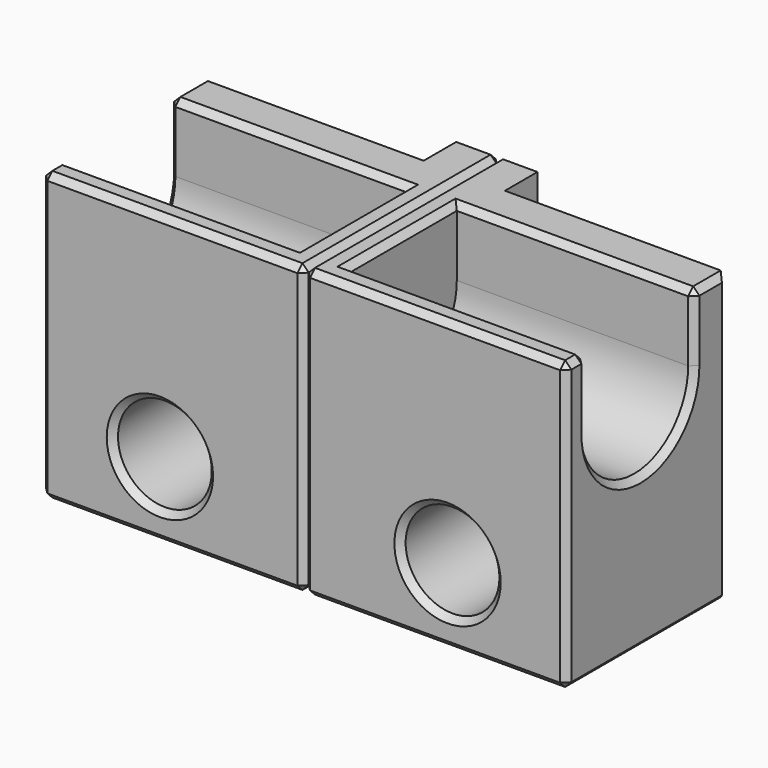
from build123d import *

# Parameters (mm, degrees)
F6_R      = 7.5
F6_R_2    = 4
F6_W      = 4
F6_H      = 4
F7_DEPTH  = 29.6
F8_DEPTH  = 2.5
F9_DEPTH  = 10
F10_DEPTH = 2.5
F12_DEPTH = 38
F14_W     = 7.5
F14_H     = 20
F15_DEPTH = 2.5
F16_R     = 7.5
F16_R_2   = 4
F17_DEPTH = 21.6
F18_SIZE  = 1


with BuildPart() as f7:
    # F6 (on Front) → F7 (new body)
    with BuildSketch(Plane.XZ):
        Polygon((0, -12), (-19, -12), (-19, -34), (0, -34), (15, -34), (15, -12), align=None)
        with Locations((0, -26)):
            Circle(F6_R, mode=Mode.SUBTRACT)
        Polygon((15, 8), (0, 8), (-19, 8), (-19, -12), (0, -12), (15, -12), align=None)
        Circle(F6_R_2, mode=Mode.SUBTRACT)
        with Locations((0, -26)):
            Circle(F6_R)
        with Locations((0, -26)):
            Circle(F6_R_2, mode=Mode.SUBTRACT)
        Polygon((-19, -12), (-19, 8), (-23, 8), (-23, -34), (-19, -34), align=None)
        Polygon((19, 8), (15, 8), (15, -12), (15, -34), (19, -34), align=None)
        Polygon((0, -34), (-19, -34), (-19, -38), (15, -38), (15, -34), align=None)
        Circle(F6_R_2)
        with Locations((-21, -36)):
            Rectangle(F6_W, F6_H)
        with Locations((17, -36)):
            Rectangle(F6_W, F6_H)
    extrude(amount=F7_DEPTH)

    # F6 (on Front) → F8 (join)
    with BuildSketch(Plane.XZ):
        Polygon((15, 8), (0, 8), (-19, 8), (-19, -12), (0, -12), (15, -12), align=None)
        Circle(F6_R_2, mode=Mode.SUBTRACT)
        Circle(F6_R_2)
    extrude(amount=-F8_DEPTH)

    # F6 (on Front) → F9 (join)
    with BuildSketch(Plane.XZ):
        Polygon((-19, -12), (-19, 8), (-23, 8), (-23, -34), (-19, -34), align=None)
        with Locations((-21, -36)):
            Rectangle(F6_W, F6_H)
    extrude(amount=-F9_DEPTH)

    # F6 (on Front) → F10 (join)
    with BuildSketch(Plane.XZ):
        Polygon((19, 8), (15, 8), (15, -12), (15, -34), (19, -34), align=None)
        with Locations((17, -36)):
            Rectangle(F6_W, F6_H)
    extrude(amount=-F10_DEPTH)

    # F11 (on face) → F12 (cut)
    with BuildSketch(Plane.YZ.offset(19)):
        with BuildLine():
            Line((-25.6, 8), (-25.6, -2.8))
            ThreePointArc((-25.6, -2.8), (-14.8, -13.6), (-4, -2.8))
            Line((-4, -2.8), (-4, 8))
            Line((-4, 8), (-25.6, 8))
        make_face()
    extrude(amount=-F12_DEPTH, mode=Mode.SUBTRACT)

    # F13: union 

    # F14 (on face) → F15 (join)
    with BuildSketch(Plane.YZ.offset(-19)):
        with Locations((6.25, -2)):
            Rectangle(F14_W, F14_H)
    extrude(amount=F15_DEPTH)

    # F16 (on face) → F17 (cut)
    with BuildSketch(Plane.XZ.offset(29.6)):
        with Locations((0, -26)):
            Circle(F16_R)
        with Locations((0, -26)):
            Circle(F16_R_2, mode=Mode.SUBTRACT)
    extrude(amount=-F17_DEPTH, mode=Mode.SUBTRACT)

    # F18
    f18_edges = [f7.edges().sort_by_distance(p)[0] for p in [
        (-4, 0, -26),
        (-23, -9.8, 8),
        (-23, -29.6, -15),
        (-23, -9.8, -38),
        (-23, 10, -15),
        (-2, -29.6, 8),
        (-2, -29.6, -38),
        (19, -29.6, -15),
        (-7.5, -29.6, -26),
        (19, -13.55, -38),
        (19, 2.5, -15),
        (19, -0.75, 8),
        (19, -4, 2.6),
        (19, -14.8, -13.6),
        (19, -25.6, 2.6),
        (19, -27.6, 8),
        (-21, 10, -38),
        (-19, 10, -25),
        (-17.75, 10, -12),
        (-16.5, 10, -2),
        (-19.75, 10, 8),
        (15, 2.5, -25),
        (-4, -8, -26),
        (0, -4, 8),
        (-19, -14.8, 8),
        (0, -25.6, 8),
    ]]
    chamfer(f18_edges, length=F18_SIZE)


with BuildPart() as f19_1:
    # F19: instance of F7
    add(f7.part.mirror(Plane(origin=(-23, -9.8, -15), x_dir=(0, -1, 0), z_dir=(-1, 0, 0))))


solid = Compound([f7.part, f19_1.part])
